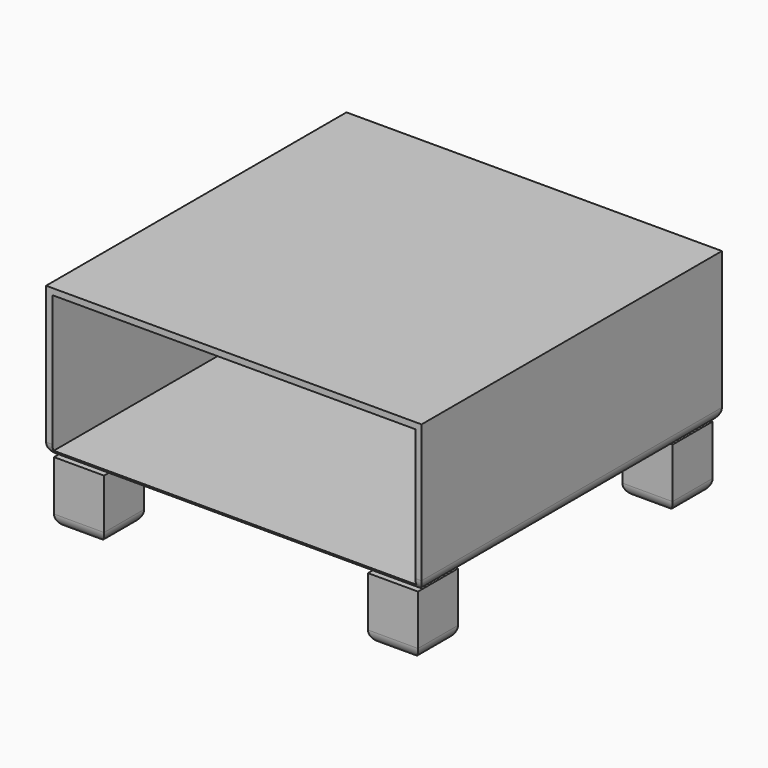
from build123d import *

# Parameters (mm, degrees)
F0_W        = 20
F0_H        = 20
F1_DEPTH    = 25
F2_W        = 150
F2_H        = 150
F3_DEPTH    = 60
F4_T        = -2.5
F5_R        = 5
F5_2_R      = 5
F5_3_R      = 5
F5_4_R      = 5
F6_T1_DEPTH = 175
F6_T3_DEPTH = 175


# Not quite as in the source:
# - a fillet or chamfer that OpenCascade refuses, or shapes differently, is made with other operations: its cross-section is extruded or revolved along the edge and cut away or added


with BuildPart() as f1:
    # F0 (on Top) → F1 (new body)
    with BuildSketch(Plane.XY):
        with Locations((-62.7156771406, 63.3284281388)):
            Rectangle(F0_W, F0_H)
    extrude(amount=-F1_DEPTH)

    # F5#4
    f5_4_edges = [f1.edges().sort_by_distance(p)[0] for p in [
        (-62.715677, 73.328428, -25),
        (-72.715677, 63.328428, -25),
        (-62.715677, 53.328428, -25),
        (-52.715677, 63.328428, -25),
    ]]
    fillet(f5_4_edges, radius=F5_4_R)


with BuildPart() as f1b:
    # F0 (on Top) → F1, piece 2 (new body)
    with BuildSketch(Plane.XY):
        with Locations((-62.7156771406, -63.7548786509)):
            Rectangle(F0_W, F0_H)
    extrude(amount=-F1_DEPTH)

    # F5
    f5_edges = [f1b.edges().sort_by_distance(p)[0] for p in [
        (-62.715677, -53.754879, -25),
        (-72.715677, -63.754879, -25),
        (-62.715677, -73.754879, -25),
        (-52.715677, -63.754879, -25),
    ]]
    fillet(f5_edges, radius=F5_R)


with BuildPart() as f1c:
    # F0 (on Top) → F1, piece 3 (new body)
    with BuildSketch(Plane.XY):
        with Locations((62.7009654807, 63.3284281388)):
            Rectangle(F0_W, F0_H)
    extrude(amount=-F1_DEPTH)

    # F5#3
    f5_3_edges = [f1c.edges().sort_by_distance(p)[0] for p in [
        (52.700965, 63.328428, -25),
        (62.700965, 53.328428, -25),
        (72.700965, 63.328428, -25),
        (62.700965, 73.328428, -25),
    ]]
    fillet(f5_3_edges, radius=F5_3_R)


with BuildPart() as f1d:
    # F0 (on Top) → F1, piece 4 (new body)
    with BuildSketch(Plane.XY):
        with Locations((62.7009654807, -63.7548786509)):
            Rectangle(F0_W, F0_H)
    extrude(amount=-F1_DEPTH)

    # F5#2
    f5_2_edges = [f1d.edges().sort_by_distance(p)[0] for p in [
        (52.700965, -63.754879, -25),
        (62.700965, -73.754879, -25),
        (72.700965, -63.754879, -25),
        (62.700965, -53.754879, -25),
    ]]
    fillet(f5_2_edges, radius=F5_2_R)


with BuildPart() as f3:
    # F2 (on Top) → F3 (new body)
    with BuildSketch(Plane.XY):
        with Locations((-3.77863e-05, 0.1337043941)):
            Rectangle(F2_W, F2_H)
    extrude(amount=F3_DEPTH)

    # F4
    f4_openings = [f3.faces().sort_by_distance(p)[0] for p in [
        (-3.8e-05, -74.866296, 30),
    ]]
    offset(amount=F4_T, openings=f4_openings)

    # F6: fillet of radius 5 on 4 edges, made by hand

    # F6_s2 → F6_t1 (cut)
    with BuildSketch(Plane.YZ.offset(-87.5000377863)):
        with BuildLine():
            ThreePointArc((75.1337043941, 5), (73.6692383, 1.4644660941), (70.1337043941, 0))
            Line((70.1337043941, 0), (75.1337043941, 0))
            Line((75.1337043941, 0), (75.1337043941, 5))
        make_face()
        with BuildLine():
            ThreePointArc((-69.8662956059, 0), (-73.4018295118, 1.4644660941), (-74.8662956059, 5))
            Line((-74.8662956059, 5), (-74.8662956059, 0))
            Line((-74.8662956059, 0), (-69.8662956059, 0))
        make_face()
    extrude(amount=F6_T1_DEPTH, mode=Mode.SUBTRACT)

    # F6_s4 → F6_t3 (cut)
    with BuildSketch(Plane.XZ.offset(-87.6337043941)):
        with BuildLine():
            ThreePointArc((-75.0000377863, 5), (-73.5355716923, 1.4644660941), (-70.0000377863, 0))
            Line((-70.0000377863, 0), (-75.0000377863, 0))
            Line((-75.0000377863, 0), (-75.0000377863, 5))
        make_face()
        with BuildLine():
            ThreePointArc((74.9999622137, 5), (73.5354961196, 1.4644660941), (69.9999622137, 0))
            Line((69.9999622137, 0), (74.9999622137, 0))
            Line((74.9999622137, 0), (74.9999622137, 5))
        make_face()
    extrude(amount=F6_T3_DEPTH, mode=Mode.SUBTRACT)


solid = Compound([f1.part, f1b.part, f1c.part, f1d.part, f3.part])
